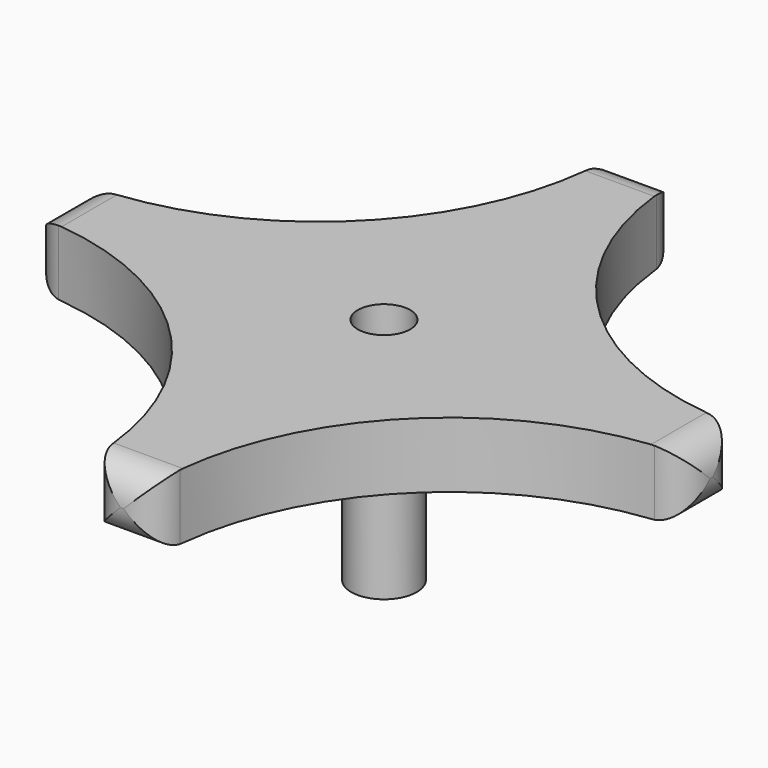
from build123d import *

# Parameters (mm, degrees)
F1_DEPTH = 10
F2_R     = 2
F3_DEPTH = 10
F2_R_2   = 4
F4_DEPTH = 5
F5_R     = 4.99999
F6_R     = 5
F6_R_2   = 2
F7_DEPTH = 25


# Not quite as in the source:
# - a fillet or chamfer is up to 0.001 mm smaller than in the source, because OpenCascade refuses the exact size


with BuildPart() as f1:
    # F0 (on Top) → F1 (new body)
    with BuildSketch(Plane.XY):
        with BuildLine():
            ThreePointArc((-50, -5), (-18.1801948466, -18.1801948466), (-5, -50))
            Line((-5, -50), (5, -50))
            ThreePointArc((5, -50), (18.1801948466, -18.1801948466), (50, -5))
            Line((50, -5), (50, 5))
            ThreePointArc((50, 5), (18.1801948466, 18.1801948466), (5, 50))
            Line((5, 50), (-5, 50))
            ThreePointArc((-5, 50), (-18.1801948466, 18.1801948466), (-50, 5))
            Line((-50, 5), (-50, -5))
        make_face()
    extrude(amount=F1_DEPTH)

    # F2 (on face) → F3 (cut, through all)
    with BuildSketch(Plane.XY.offset(10)):
        Circle(F2_R)
    extrude(amount=-F3_DEPTH, mode=Mode.SUBTRACT)

    # F2 (on face) → F4 (cut)
    with BuildSketch(Plane.XY.offset(10)):
        Circle(F2_R_2)
        Circle(F2_R, mode=Mode.SUBTRACT)
    extrude(amount=-F4_DEPTH, mode=Mode.SUBTRACT)

    # F5 (radius 5 in the source; OpenCascade refuses exactly that, so slightly less here)
    f5_edges = [f1.edges().sort_by_distance(p)[0] for p in [
        (5, 50, 5),
        (-5, 50, 5),
        (0, 50, 0),
        (0, 50, 10),
        (-50, 5, 5),
        (-50, -5, 5),
        (-50, 0, 0),
        (-50, 0, 10),
        (-5, -50, 5),
        (5, -50, 5),
        (0, -50, 0),
        (0, -50, 10),
        (50, -5, 5),
        (50, 5, 5),
        (50, 0, 0),
        (50, 0, 10),
    ]]
    fillet(f5_edges, radius=F5_R)

    # F6 (on face) → F7 (join)
    with BuildSketch(Plane(origin=(0, 0, 0), x_dir=(1, 0, 0), z_dir=(0, 0, -1))):
        Circle(F6_R)
        Circle(F6_R_2, mode=Mode.SUBTRACT)
    extrude(amount=F7_DEPTH)


solid = f1.part
